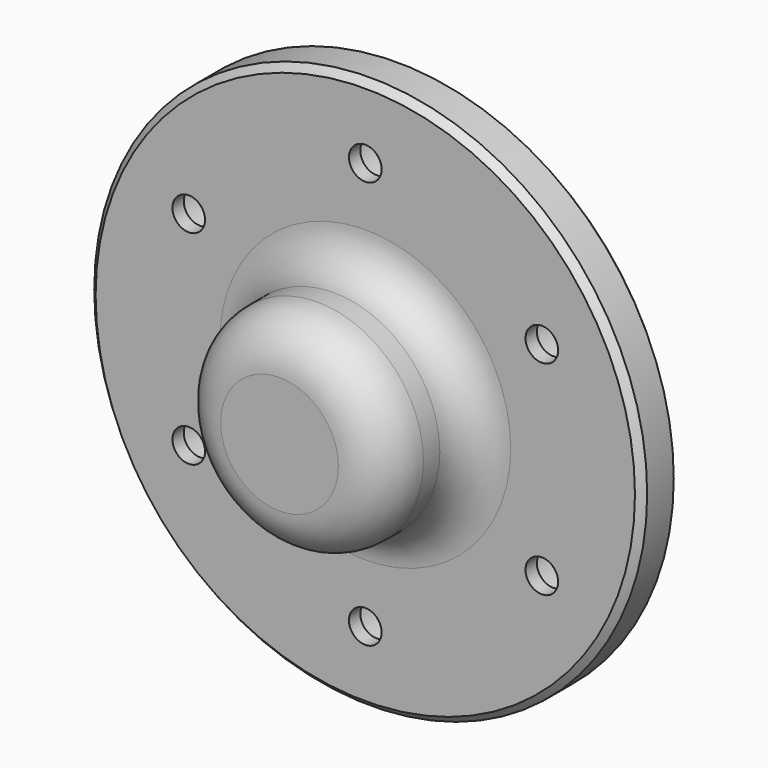
from build123d import *

# Parameters (mm, degrees)
F4_D            = 6.096
F4_CBORE_D      = 12.192
F4_CBORE_DEPTH  = 6.096
F4_COPIES_COUNT = 6
F5_R            = 7.3585229381
F6_R            = 8.8302275257
F7_SIZE         = 1.27


# Not quite as in the source:
# - a pattern or mirror of a feature is missing from the dataset's text; its kind, count and spacing are read off the source's solid


with BuildPart() as f2:
    # F1 (on Top) → F2 (revolve)
    with BuildSketch(Plane.XY):
        Polygon((0, 23.1950208545), (0, 0), (19.8225509375, 0), (19.8225509375, 20.0292905793), (51.67459324, 20.0292905793), (51.67459324, 28.776070103), (10.3429872543, 28.776070103), (10.3429872543, 23.1950208545), align=None)
    revolve(axis=Axis((0, 11.5975104272, 0), (0, -1, 0)))

    # F4 (through all)
    with Locations(Plane(origin=(0, 28.776070103, 0), x_dir=(-1, 0, 0), z_dir=(0, 1, 0))):
        with Locations((0, -38.1)):
            f4 = CounterBoreHole(F4_D / 2, F4_CBORE_D / 2, F4_CBORE_DEPTH)

    # F4_copies: F4 ×6 about axis
    f4_copies_axis = Axis((0, 0, 0), (0, 1, 0))
    for i in range(1, F4_COPIES_COUNT):
        add(f4.rotate(f4_copies_axis, i * 360 / F4_COPIES_COUNT), mode=Mode.SUBTRACT)

    # F5
    f5_edges = [f2.edges().sort_by_distance(p)[0] for p in [
        (-19.822551, 20.029291, 0),
    ]]
    fillet(f5_edges, radius=F5_R)

    # F6
    f6_edges = [f2.edges().sort_by_distance(p)[0] for p in [
        (-19.822551, 0, 0),
    ]]
    fillet(f6_edges, radius=F6_R)

    # F7
    f7_edges = [f2.edges().sort_by_distance(p)[0] for p in [
        (-51.674593, 20.029291, 0),
        (-51.674593, 28.77607, 0),
    ]]
    chamfer(f7_edges, length=F7_SIZE)


solid = f2.part
